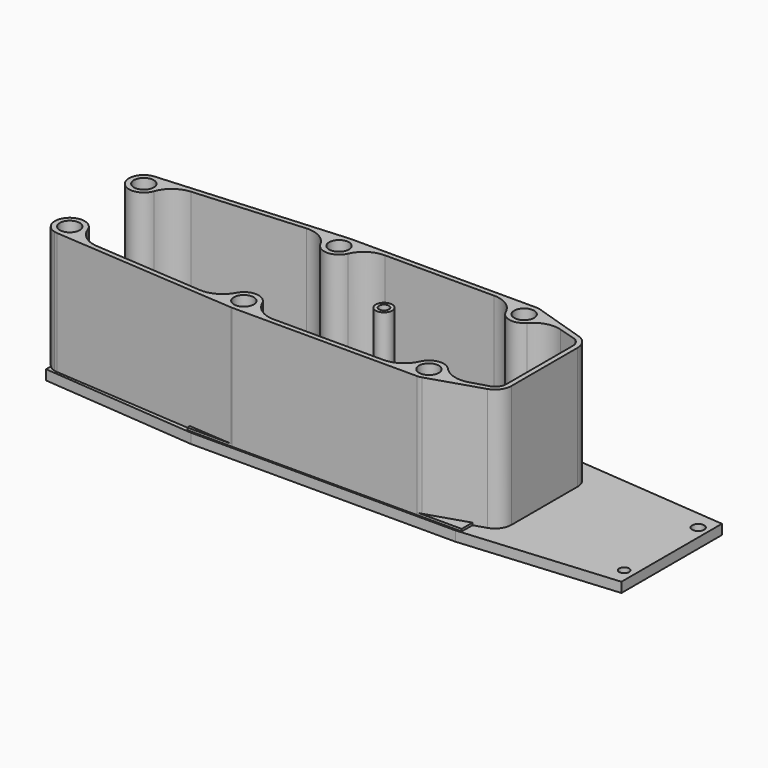
from build123d import *

# Parameters (mm, degrees)
F0_R          = 1.5
F0_R_2        = 2.7
F0_R_3        = 1.819408366
F1_DEPTH      = 3
F0_R_4        = 1.3
F2_DEPTH      = 6
F2_DEPTH_BACK = 3
F3_DEPTH      = 6
F3_DEPTH_BACK = 3
F4_DEPTH      = 6
F4_DEPTH_BACK = 3
F5_DEPTH      = 6
F5_DEPTH_BACK = 3
F6_W          = 83
F6_H          = 45
F6_R          = 1.5
F6_R_2        = 3
F6_W_2        = 10
F6_H_2        = 10
F6_W_3        = 6.5
F6_H_3        = 6.5
F7_DEPTH      = 0.7
F8_DEPTH      = 3
F9_DEPTH      = 3
F10_R         = 2.5
F10_R_2       = 1.5
F11_DEPTH     = 37
F12_R         = 3
F13_DEPTH     = 37


with BuildPart() as f1:
    # F0 (on Top) → F1 (new body)
    with BuildSketch(Plane.XY):
        Polygon((40, 23), (-40, 23), (-87.0266780257, 19), (-87.0266780257, -19), (-40, -23), (40, -23), (87.0266780257, -19), (87.0266780257, 19), align=None)
        with Locations((-83.8569601751, -14)):
            Circle(F0_R, mode=Mode.SUBTRACT)
        with Locations((-28, -18)):
            Circle(F0_R, mode=Mode.SUBTRACT)
        with Locations((-15.3, -15.03)):
            Circle(F0_R_2, mode=Mode.SUBTRACT)
        with Locations((28, -18)):
            Circle(F0_R, mode=Mode.SUBTRACT)
        with Locations((15.3, -15.03)):
            Circle(F0_R_2, mode=Mode.SUBTRACT)
        with Locations((83.8569601751, -14)):
            Circle(F0_R, mode=Mode.SUBTRACT)
        with Locations((-83.8569601751, 14)):
            Circle(F0_R, mode=Mode.SUBTRACT)
        with Locations((-15.3, 15.03)):
            Circle(F0_R_2, mode=Mode.SUBTRACT)
        with Locations((-28, 18)):
            Circle(F0_R, mode=Mode.SUBTRACT)
        with Locations((15.3, 15.03)):
            Circle(F0_R_2, mode=Mode.SUBTRACT)
        with Locations((28, 18)):
            Circle(F0_R, mode=Mode.SUBTRACT)
        with Locations((83.8569601751, 14)):
            Circle(F0_R_3, mode=Mode.SUBTRACT)
    extrude(amount=-F1_DEPTH)

    # F0 (on Top) → F2 (join, two sides)
    with BuildSketch(Plane.XY) as f2_sk:
        with Locations((-15.3, 15.03)):
            Circle(F0_R_2)
        with Locations((-15.3, 15.03)):
            Circle(F0_R_4, mode=Mode.SUBTRACT)
    extrude(amount=F2_DEPTH)
    extrude(f2_sk.sketch, amount=-F2_DEPTH_BACK)

    # F0 (on Top) → F3 (join, two sides)
    with BuildSketch(Plane.XY) as f3_sk:
        with Locations((15.3, 15.03)):
            Circle(F0_R_2)
        with Locations((15.3, 15.03)):
            Circle(F0_R_4, mode=Mode.SUBTRACT)
    extrude(amount=F3_DEPTH)
    extrude(f3_sk.sketch, amount=-F3_DEPTH_BACK)

    # F0 (on Top) → F4 (join, two sides)
    with BuildSketch(Plane.XY) as f4_sk:
        with Locations((-15.3, -15.03)):
            Circle(F0_R_2)
        with Locations((-15.3, -15.03)):
            Circle(F0_R_4, mode=Mode.SUBTRACT)
    extrude(amount=F4_DEPTH)
    extrude(f4_sk.sketch, amount=-F4_DEPTH_BACK)

    # F0 (on Top) → F5 (join, two sides)
    with BuildSketch(Plane.XY) as f5_sk:
        with Locations((15.3, -15.03)):
            Circle(F0_R_2)
        with Locations((15.3, -15.03)):
            Circle(F0_R_4, mode=Mode.SUBTRACT)
    extrude(amount=F5_DEPTH)
    extrude(f5_sk.sketch, amount=-F5_DEPTH_BACK)


with BuildPart() as f7:
    # F6 (on Top) → F7 (new body)
    with BuildSketch(Plane.XY):
        Rectangle(F6_W, F6_H)
        with Locations((-28, -18)):
            Circle(F6_R, mode=Mode.SUBTRACT)
        with Locations((-15.3, -15.03)):
            Circle(F6_R_2, mode=Mode.SUBTRACT)
        with Locations((15.3, -15.03)):
            Circle(F6_R_2, mode=Mode.SUBTRACT)
        with Locations((28, -18)):
            Circle(F6_R, mode=Mode.SUBTRACT)
        with Locations((-28, 18)):
            Circle(F6_R, mode=Mode.SUBTRACT)
        with Locations((-15.3, 15.03)):
            Circle(F6_R_2, mode=Mode.SUBTRACT)
        Rectangle(F6_W_2, F6_H_2, mode=Mode.SUBTRACT)
        with Locations((11.75, 0)):
            Rectangle(F6_W_3, F6_H_3, mode=Mode.SUBTRACT)
        with Locations((20.75, 0)):
            Rectangle(F6_W_3, F6_H_3, mode=Mode.SUBTRACT)
        with Locations((15.3, 15.03)):
            Circle(F6_R_2, mode=Mode.SUBTRACT)
        with Locations((28, 18)):
            Circle(F6_R, mode=Mode.SUBTRACT)
    extrude(amount=F7_DEPTH)

    # F6 (on Top) → F8 (join)
    with BuildSketch(Plane.XY):
        with Locations((11.75, 0)):
            Rectangle(F6_W_3, F6_H_3)
    extrude(amount=F8_DEPTH)

    # F6 (on Top) → F9 (join)
    with BuildSketch(Plane.XY):
        with Locations((20.75, 0)):
            Rectangle(F6_W_3, F6_H_3)
    extrude(amount=F9_DEPTH)


with BuildPart() as f11:
    # F10 (on Top) → F11 (new body)
    with BuildSketch(Plane.XY):
        Circle(F10_R)
        Circle(F10_R_2, mode=Mode.SUBTRACT)
    extrude(amount=F11_DEPTH)


with BuildPart() as f13:
    # F12 (on Top) → F13 (new body)
    with BuildSketch(Plane.XY):
        with BuildLine():
            ThreePointArc((-39.6414619684, 20.1740200639), (-35.1775366862, 19.1836223263), (-31.9852120229, 15.9100035568))
            ThreePointArc((-31.9852120229, 15.9100035568), (-27.8391829885, 13.502874486), (-23.8756818745, 16.2))
            ThreePointArc((-23.8756818745, 16.2), (-20.9253412227, 19.6932802123), (-16.5435607626, 21))
            Line((-16.5435607626, 21), (16.5435607626, 21))
            ThreePointArc((16.5435607626, 21), (20.9253412227, 19.6932802123), (23.8756818745, 16.2))
            ThreePointArc((23.8756818745, 16.2), (27.2788858407, 13.5581541709), (31.3430629249, 14.9877034873))
            ThreePointArc((31.3430629249, 14.9877034873), (35.1356458892, 17.3380108085), (39.5971998807, 17.291470229))
            Line((39.5971998807, 17.291470229), (45.1684511965, 15.6104741628))
            ThreePointArc((45.1684511965, 15.6104741628), (46.5526259047, 14.3212182344), (47.0637859721, 12.5))
            Line((47.0637859721, 12.5), (47.0637859721, -12.5))
            ThreePointArc((47.0637859721, -12.5), (46.170734794, -14.8353410543), (43.9473186349, -15.9789226345))
            Line((43.9473186349, -15.9789226345), (39.5971998807, -17.291470229))
            ThreePointArc((39.5971998807, -17.291470229), (35.1356458892, -17.3380108085), (31.3430629249, -14.9877034873))
            ThreePointArc((31.3430629249, -14.9877034873), (27.2788858407, -13.5581541709), (23.8756818745, -16.2))
            ThreePointArc((23.8756818745, -16.2), (20.9253412227, -19.6932802123), (16.5435607626, -21))
            Line((16.5435607626, -21), (-16.5435607626, -21))
            ThreePointArc((-16.5435607626, -21), (-20.9253412227, -19.6932802123), (-23.8756818745, -16.2))
            ThreePointArc((-23.8756818745, -16.2), (-27.8391829885, -13.502874486), (-31.9852120229, -15.9100035568))
            ThreePointArc((-31.9852120229, -15.9100035568), (-35.1775366862, -19.1836223263), (-39.6414619684, -20.1740200639))
            Line((-39.6414619684, -20.1740200639), (-72.6440696352, -17.8106542406))
            ThreePointArc((-72.6440696352, -17.8106542406), (-76.921320662, -16.1942878659), (-79.614605295, -12.4991918605))
            ThreePointArc((-79.614605295, -12.4991918605), (-87.1459536038, -10.9287588461), (-85.0641073106, -18.3350658349))
            Line((-85.0641073106, -18.3350658349), (-84.1783887465, -18.4885057284))
            Line((-84.1783887465, -18.4885057284), (-28.3214285714, -22.4885057284))
            ThreePointArc((-28.3214285714, -22.4885057284), (-28.1608170115, -22.497125514), (-28, -22.5))
            Line((-28, -22.5), (28, -22.5))
            ThreePointArc((28, -22.5), (28.693358688, -22.4462628948), (29.3701577809, -22.286334991))
            Line((29.3701577809, -22.286334991), (45.0861835065, -17.2625944345))
            ThreePointArc((45.0861835065, -17.2625944345), (47.6018540542, -15.4485600153), (48.5637859721, -12.5))
            Line((48.5637859721, -12.5), (48.5637859721, 12.5))
            ThreePointArc((48.5637859721, 12.5), (47.6018540542, 15.4485600153), (45.0861835065, 17.2625944345))
            Line((45.0861835065, 17.2625944345), (29.3701577809, 22.286334991))
            ThreePointArc((29.3701577809, 22.286334991), (28.693358688, 22.4462628948), (28, 22.5))
            Line((28, 22.5), (-28, 22.5))
            ThreePointArc((-28, 22.5), (-28.1608170115, 22.497125514), (-28.3214285714, 22.4885057284))
            Line((-28.3214285714, 22.4885057284), (-84.1783887465, 18.4885057284))
            ThreePointArc((-84.1783887465, 18.4885057284), (-87.4362598177, 11.272617726), (-79.614605295, 12.4991918605))
            ThreePointArc((-79.614605295, 12.4991918605), (-76.921320662, 16.1942878659), (-72.6440696352, 17.8106542406))
            Line((-72.6440696352, 17.8106542406), (-39.6414619684, 20.1740200639))
        make_face()
        with Locations((-83.8569601751, -14)):
            Circle(F12_R, mode=Mode.SUBTRACT)
        with Locations((-28, -18)):
            Circle(F12_R, mode=Mode.SUBTRACT)
        with Locations((28, -18)):
            Circle(F12_R, mode=Mode.SUBTRACT)
        with Locations((-83.8569601751, 14)):
            Circle(F12_R, mode=Mode.SUBTRACT)
        with BuildLine():
            Line((-82.8338199445, 18.3821437754), (-84.1783887465, 18.4885057284))
            ThreePointArc((-84.1783887465, 18.4885057284), (-83.5020967796, 18.4859861759), (-82.8338199445, 18.3821437754))
        make_face(mode=Mode.SUBTRACT)
        with Locations((-28, 18)):
            Circle(F12_R, mode=Mode.SUBTRACT)
        with Locations((28, 18)):
            Circle(F12_R, mode=Mode.SUBTRACT)
        with BuildLine():
            ThreePointArc((-82.8338199445, 18.3821437754), (-83.5020967796, 18.4859861759), (-84.1783887465, 18.4885057284))
            Line((-84.1783887465, 18.4885057284), (-82.8338199445, 18.3821437754))
        make_face()
        with BuildLine():
            ThreePointArc((-85.0641073106, -18.3350658349), (-84.625088988, -18.4339573889), (-84.1783887465, -18.4885057284))
            Line((-84.1783887465, -18.4885057284), (-85.0641073106, -18.3350658349))
        make_face()
    extrude(amount=F13_DEPTH)


solid = Compound([f1.part, f7.part, f11.part, f13.part])
